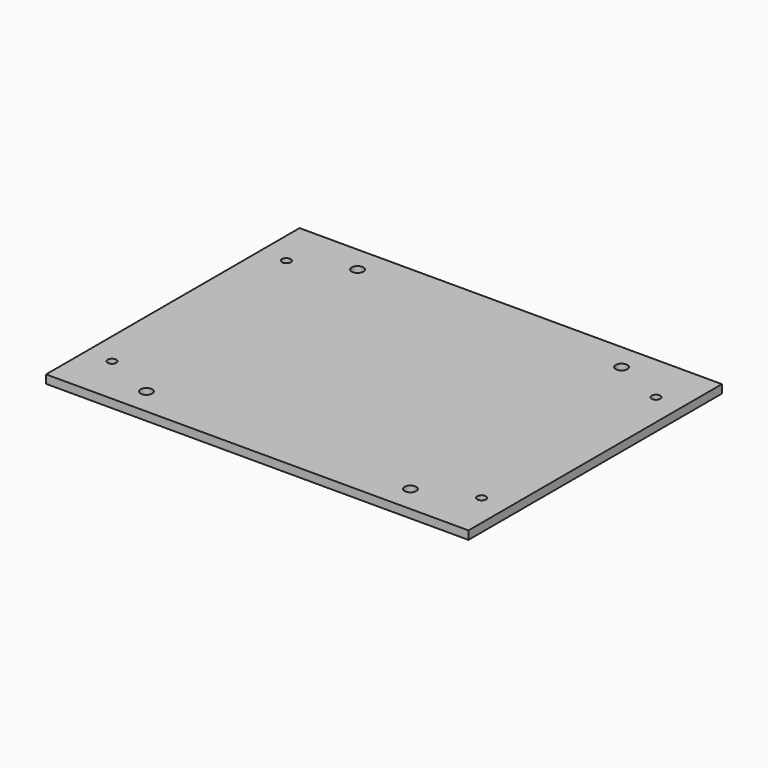
from build123d import *

# Parameters (mm, degrees)
F0_W     = 160
F0_H     = 120
F0_R     = 2.2
F0_R_2   = 1.65
F1_DEPTH = 3.175


# Not quite as in the source:
# - a length typed as a fraction of an inch, garbled in the dataset ("3 / 203.2 mm" for 3/8 in), is restored


with BuildPart() as f1:
    # F0 (on Top) → F1 (new body)
    with BuildSketch(Plane.XY):
        Rectangle(F0_W, F0_H)
        with Locations((-50, -50)):
            Circle(F0_R, mode=Mode.SUBTRACT)
        with Locations((-70, -41.26)):
            Circle(F0_R_2, mode=Mode.SUBTRACT)
        with Locations((50, -50)):
            Circle(F0_R, mode=Mode.SUBTRACT)
        with Locations((70, -41.26)):
            Circle(F0_R_2, mode=Mode.SUBTRACT)
        with Locations((-70, 41.26)):
            Circle(F0_R_2, mode=Mode.SUBTRACT)
        with Locations((-50, 50)):
            Circle(F0_R, mode=Mode.SUBTRACT)
        with Locations((70, 41.26)):
            Circle(F0_R_2, mode=Mode.SUBTRACT)
        with Locations((50, 50)):
            Circle(F0_R, mode=Mode.SUBTRACT)
    extrude(amount=F1_DEPTH)


solid = f1.part
